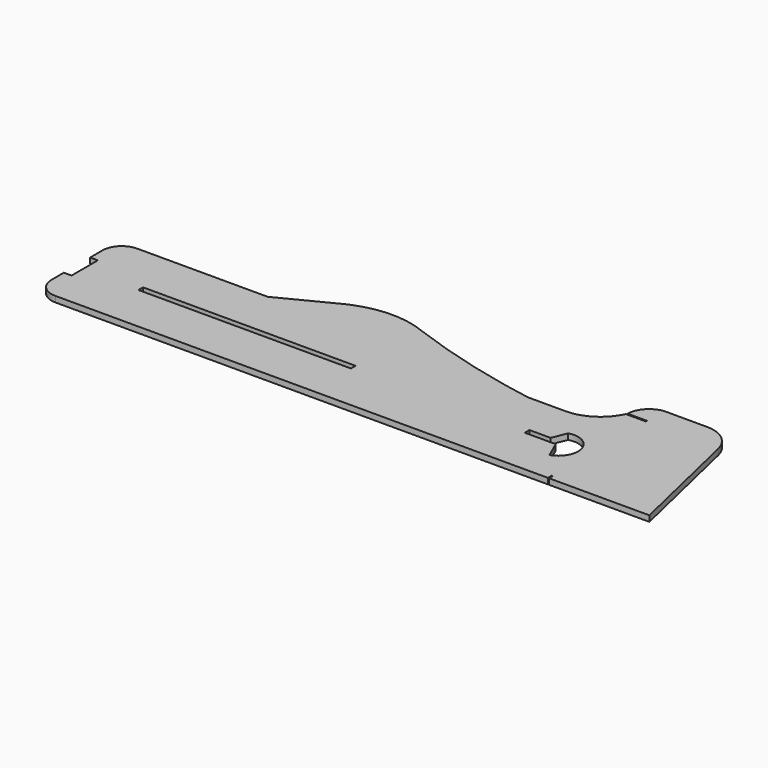
from build123d import *

# Parameters (mm, degrees)
F1_DEPTH = 6


with BuildPart() as f1:
    # F0 (on Top) → F1 (new body)
    with BuildSketch(Plane.XY):
        Polygon((-297.5, -55), (-297.5, -75), (-162.5, -75), (-162.5, -25), (-251.5, -25), (-251.5, -22), (-309.5, -22), (-309.5, -39), (-317.5, -39), (-317.5, -55), align=None)
        with BuildLine():
            ThreePointArc((-317.5, -55), (-311.6421356237, -69.1421356237), (-297.5, -75))
            Line((-297.5, -75), (-297.5, -55))
            Line((-297.5, -55), (-317.5, -55))
        make_face()
        with BuildLine():
            Line((-162.5, -25), (-162.5, -75))
            Line((-162.5, -75), (212.5, -75))
            Line((212.5, -75), (212.5, -70))
            Line((212.5, -70), (212.5, -22))
            Line((212.5, -22), (202.5606023011, -22))
            ThreePointArc((202.5606023011, -22), (199.1728742742, -34.9388939069), (188.5, -43))
            Line((188.5, -43), (180.5, -43))
            Line((180.5, -43), (180.5, -25))
            Line((180.5, -25), (148.5, -25))
            Line((148.5, -25), (148.5, -22))
            Line((148.5, -22), (-31.5, -22))
            Line((-31.5, -22), (-31.5, -25))
            Line((-31.5, -25), (-162.5, -25))
        make_face()
        with BuildLine():
            Line((213.5, -70), (213.5, -75))
            Line((213.5, -75), (317.5, -75))
            Line((317.5, -75), (288.1807403902, 50.6539697565))
            ThreePointArc((288.1807403902, 50.6539697565), (277.083392323, 68.1740192438), (257.5, 75))
            Line((257.5, 75), (212.5, 75))
            Line((212.5, 75), (212.5, 53))
            Line((212.5, 53), (212.5, 51.5))
            Line((212.5, 51.5), (212.5, -22))
            Line((212.5, -22), (212.5, -70))
            Line((212.5, -70), (213.5, -70))
        make_face()
        Polygon((-317.5, 11), (-317.5, -5), (-309.5, -5), (-309.5, -22), (-251.5, -22), (-251.5, -19), (-162.5, -19), (-162.5, 31), (-297.5, 31), (-297.5, 11), align=None)
        with BuildLine():
            Line((202.5606023011, -22), (212.5, -22))
            Line((212.5, -22), (212.5, 51.5))
            Line((212.5, 51.5), (191.8430768086, 51.5))
            ThreePointArc((191.8430768086, 51.5), (175.0535129869, 32.1936689306), (150.5, 25))
            Line((150.5, 25), (112.5, 25))
            Line((112.5, 25), (-107.5, 25))
            Line((-107.5, 25), (-107.5, 31))
            Line((-107.5, 31), (-162.5, 31))
            Line((-162.5, 31), (-162.5, -19))
            Line((-162.5, -19), (-31.5, -19))
            Line((-31.5, -19), (-31.5, -22))
            Line((-31.5, -22), (148.5, -22))
            Line((148.5, -22), (148.5, -19))
            Line((148.5, -19), (170.5, -19))
            Line((170.5, -19), (170.5, -4))
            Line((170.5, -4), (176.5, -4))
            ThreePointArc((176.5, -4), (193.8141294499, -6.7978252425), (202.5606023011, -22))
        make_face()
        with BuildLine():
            ThreePointArc((-297.5, 31), (-311.6421356237, 25.1421356237), (-317.5, 11))
            Line((-317.5, 11), (-297.5, 11))
            Line((-297.5, 11), (-297.5, 31))
        make_face()
        Polygon((-107.5, 59), (-162.5, 31), (-107.5, 31), align=None)
        with BuildLine():
            Line((192.5, 53), (212.5, 53))
            Line((212.5, 53), (212.5, 75))
            ThreePointArc((212.5, 75), (198.4968622639, 67.6392161237), (192.5, 53))
        make_face()
        Polygon((180.5, -43), (188.5, -43), (180.5, -25), align=None)
        Polygon((170.5, -19), (176.5, -4), (170.5, -4), align=None)
        with BuildLine():
            Line((-107.5, 59), (-107.5, 31))
            Line((-107.5, 31), (80.5750319553, 31))
            ThreePointArc((80.5750319553, 31), (25.9745832288, 44.5374524252), (-27.5, 62))
            Line((-27.5, 62), (-27.5, 59))
            Line((-27.5, 59), (-107.5, 59))
        make_face()
        with BuildLine():
            Line((80.5750319553, 31), (-107.5, 31))
            Line((-107.5, 31), (-107.5, 25))
            Line((-107.5, 25), (112.5, 25))
            ThreePointArc((112.5, 25), (96.5060750704, 27.8327083402), (80.5750319553, 31))
        make_face()
        with BuildLine():
            ThreePointArc((-101.0171084337, 62), (-104.2866693361, 60.5607557565), (-107.5, 59))
            Line((-107.5, 59), (-27.5, 59))
            Line((-27.5, 59), (-27.5, 62))
            Line((-27.5, 62), (-101.0171084337, 62))
        make_face()
        with BuildLine():
            ThreePointArc((-27.5, 62), (-64.2585542169, 69.3734629996), (-101.0171084337, 62))
            Line((-101.0171084337, 62), (-27.5, 62))
        make_face()
    extrude(amount=F1_DEPTH)


solid = f1.part
